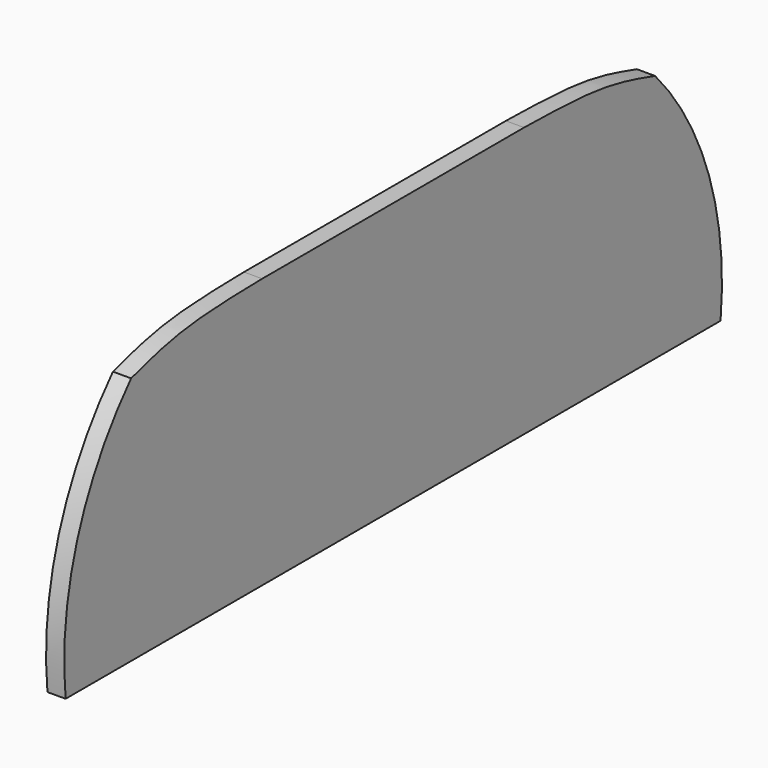
from build123d import *

# Parameters (mm, degrees)
F1_DEPTH = 25.4


with BuildPart() as f1:
    # F0 (on Right) → F1 (new body)
    with BuildSketch(Plane.YZ):
        with BuildLine():
            Line((228.6, 376.9212961197), (0, 376.9212961197))
            Line((0, 376.9212961197), (-228.6, 376.9212961197))
            add(Edge.make_bspline(
                [(-457.2753436089, 347.454816103), (-428.9132900906, 355.8432406544), (-365.8930365544, 374.4822521654), (-277.3142184262, 376.0558762636), (-228.6, 376.9212961197)],
                knots=[0, 0, 0, 0, 0.4500466426, 1, 1, 1, 1], degree=3))
            ThreePointArc((-457.2753436089, 347.454816103), (-551.68686479, 185.9850935796), (-571.5753436089, 0))
            Line((-571.5753436089, 0), (0, 0))
            Line((0, 0), (571.5753436089, 0))
            ThreePointArc((571.5753436089, 0), (551.68686479, 185.9850935796), (457.2753436089, 347.454816103))
            add(Edge.make_bspline(
                [(457.2753436089, 347.454816103), (428.9132900906, 355.8432406544), (365.8930365544, 374.4822521654), (277.3142184262, 376.0558762636), (228.6, 376.9212961197)],
                knots=[0, 0, 0, 0, 0.4500466426, 1, 1, 1, 1], degree=3))
        make_face()
    extrude(amount=F1_DEPTH)


solid = f1.part
